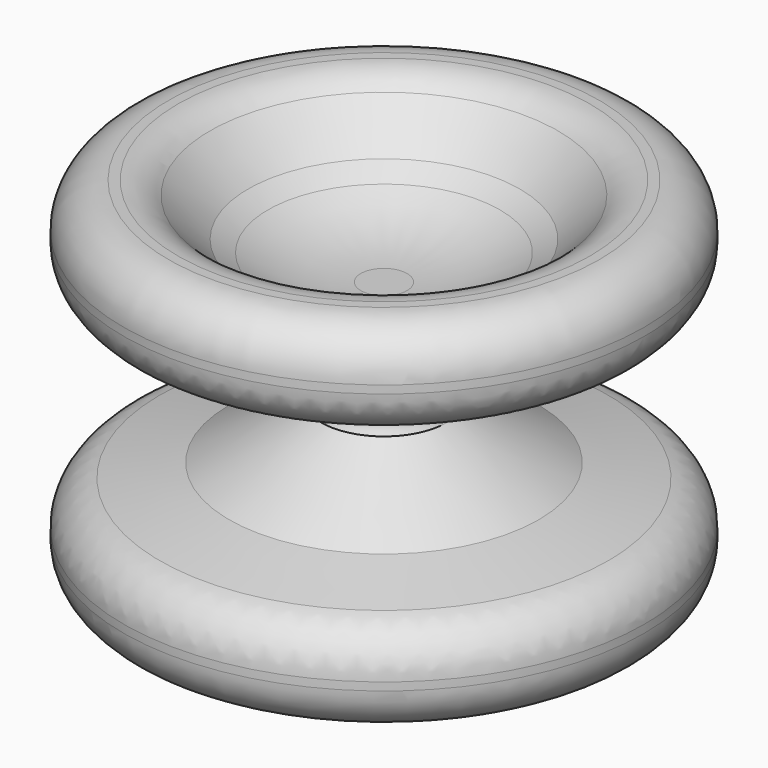
from build123d import *
from build123d import SkipClean  # not in build123d's __all__

# Parameters (mm, degrees)
F2_R = 5
F3_R = 20


# Not quite as in the source:
# - a pattern or mirror of a feature is missing from the dataset's text; its kind, count and spacing are read off the source's solid


with BuildPart() as f1:
    # F0 (on Front) → F1 (revolve)
    with BuildSketch(Plane.XZ):
        with BuildLine():
            Line((6.5, 0), (0, 0))
            Line((0, 0), (0, -10))
            Line((0, -10), (8.146820964, -10))
            Line((8.146820964, -10), (15.1208594459, -14.2111137569))
            Line((15.1208594459, -14.2111137569), (20.853179036, -20))
            Line((20.853179036, -20), (29, -20))
            Line((29, -20), (29, -10))
            Line((29, -10), (17.250610332, -7.6895967878))
            Line((17.250610332, -7.6895967878), (7, -1.5))
            ThreePointArc((7, -1.5), (6.6282917549, -0.790569415), (6.5, 0))
        make_face()
    revolve(axis=Axis((0, 0, -5), (0, 0, -1)))

    # F1_copies: F1 across plane


with BuildPart() as f1_1:
    add(f1.part, clean=False)
    with SkipClean():  # cleaning this boolean's faces spoils the solid; the shape is the same uncleaned
        add(f1.part.mirror(Plane.XY), clean=False)

    # F2
    f2_edges = [f1_1.edges().sort_by_distance(p)[0] for p in [
        (-29, 0, -10),
        (-29, 0, -20),
        (-20.853179, 0, -20),
        (-29, 0, 10),
        (-29, 0, 20),
        (-20.853179, 0, 20),
    ]]
    fillet(f2_edges, radius=F2_R)

    # F3
    f3_edges = [f1_1.edges().sort_by_distance(p)[0] for p in [
        (-8.146821, 0, -10),
        (-8.146821, 0, 10),
    ]]
    fillet(f3_edges, radius=F3_R)


solid = f1_1.part
